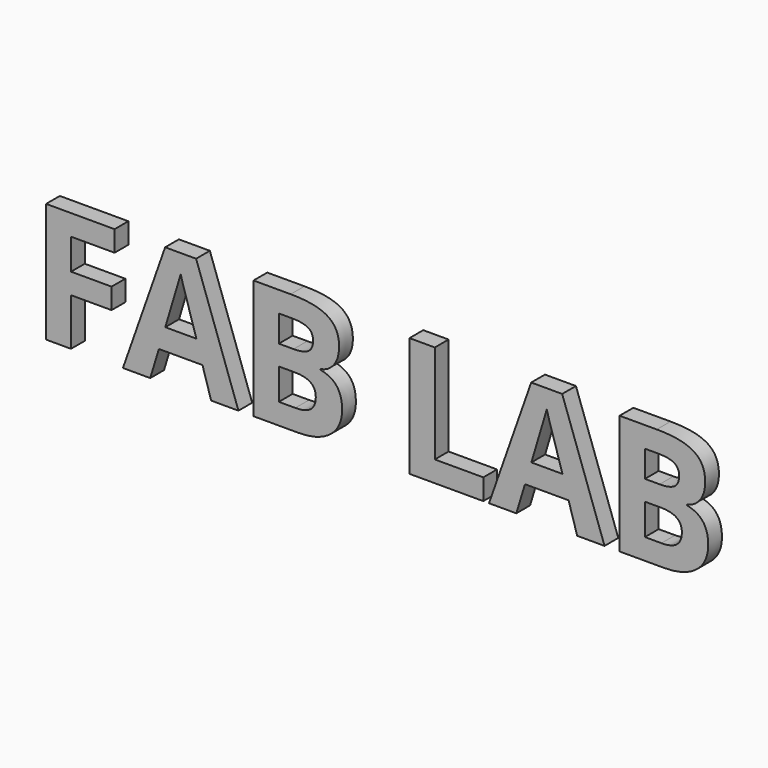
from build123d import *

# Parameters (mm, degrees)
F0_TEXT_SIZE = 243.3275036119
F1_DEPTH     = 25


# Not quite as in the source:
# - Text() gives the source's letters only with a copy of the font that has no kerning and outlines rounded to 1/6400 em; it was checked with that copy


with BuildPart() as f1:
    # F0 (on Front) → F1 (new body)
    with BuildSketch(Plane.XZ):
        with Locations((-512.6681367698, -33.2899705155)):
            Text('FAB LAB', F0_TEXT_SIZE, font='Open Sans', font_style=FontStyle.BOLD, text_align=(TextAlign.LEFT, TextAlign.BOTTOM))
    extrude(amount=F1_DEPTH)


solid = f1.part
